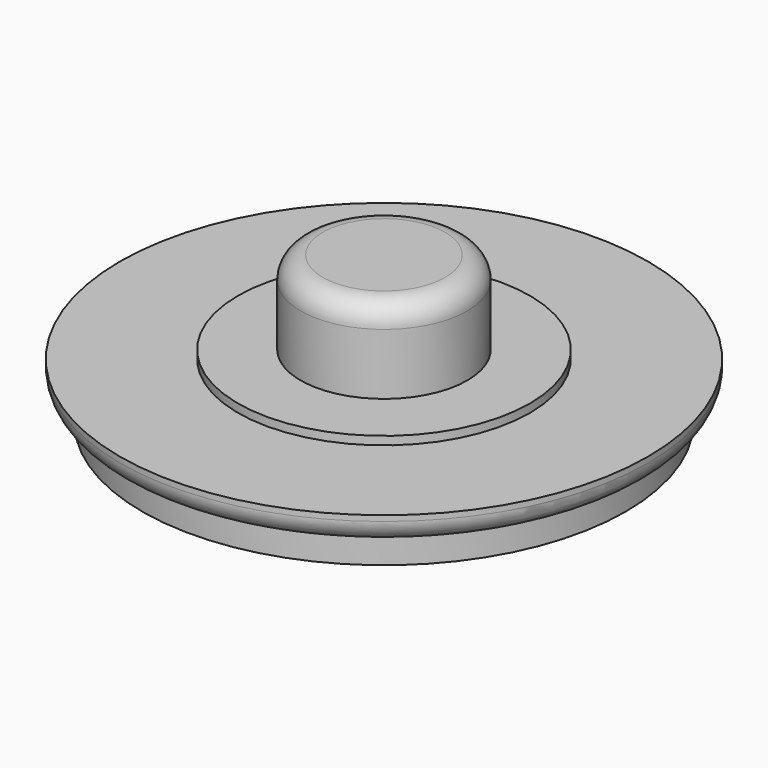
from build123d import *

# Parameters (mm, degrees)
F0_R     = 9.5
F1_DEPTH = 1
F2_R     = 3
F3_DEPTH = 3.3
F4_R     = 0.8
F5_R     = 5.25
F5_R_2   = 3
F6_DEPTH = 0.3
F7_R     = 8.7
F7_R_2   = 7.75
F7_R_3   = 6.25
F7_R_4   = 5.25
F7_R_5   = 3.75
F7_R_6   = 2.75
F8_DEPTH = 1


# Not quite as in the source:
# - a feature names something its author has since deleted; it is built from what else it names


with BuildPart() as f1:
    # F0 (on Top) → F1 (new body)
    with BuildSketch(Plane.XY):
        Circle(F0_R)
    extrude(amount=F1_DEPTH)

    # F2 (on face) → F3 (join)
    with BuildSketch(Plane.XY.offset(1)):
        Circle(F2_R)
    extrude(amount=F3_DEPTH)

    # F4
    f4_edges = [f1.edges().sort_by_distance(p)[0] for p in [
        (-9.5, 0, 0),
        (-3, 0, 4.3),
    ]]
    fillet(f4_edges, radius=F4_R)

    # F5 (on face) → F6 (join)
    with BuildSketch(Plane.XY.offset(1)):
        Circle(F5_R)
        Circle(F5_R_2, mode=Mode.SUBTRACT)
        Circle(F5_R_2)
    extrude(amount=F6_DEPTH)

    # F7 (on face) → F8 (join)
    with BuildSketch(Plane(origin=(0, 0, 0), x_dir=(1, 0, 0), z_dir=(0, 0, -1))):
        Circle(F7_R)
        Circle(F7_R_2, mode=Mode.SUBTRACT)
        Circle(F7_R_3)
        Circle(F7_R_4, mode=Mode.SUBTRACT)
        Circle(F7_R_5)
        Circle(F7_R_6, mode=Mode.SUBTRACT)
    extrude(amount=F8_DEPTH)


solid = f1.part
